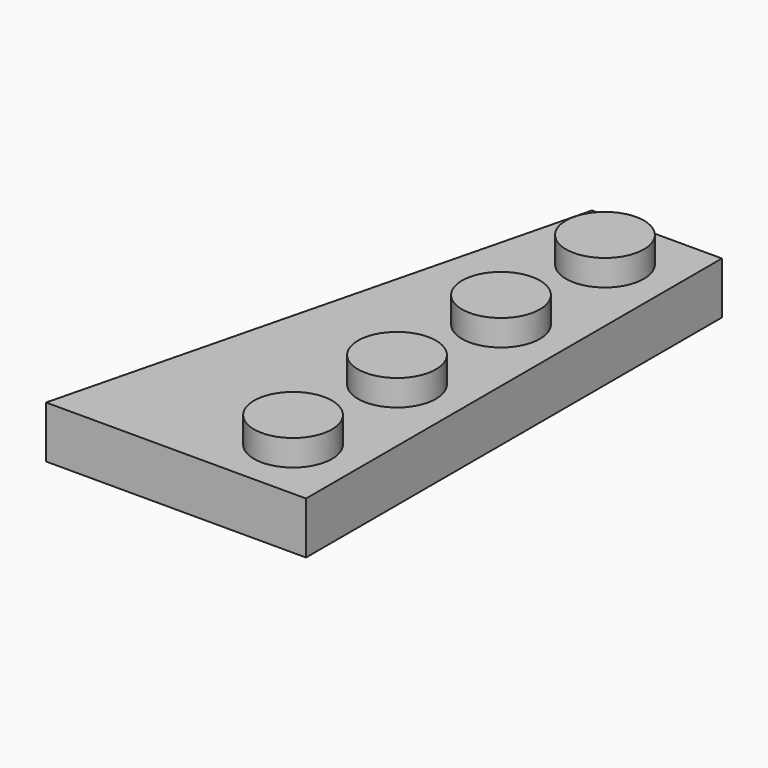
from build123d import *

# Parameters (mm, degrees)
F0_R     = 2.38125
F1_DEPTH = 3.175
F2_DEPTH = 4.7625
F3_T     = -1.5875
F4_R     = 3.175
F4_R_2   = 2.38125
F5_DEPTH = 1.5875


with BuildPart() as f1:
    # F0 (on Top) → F1 (new body)
    with BuildSketch(Plane.XY):
        Polygon((7.9375, 15.875), (0, 15.875), (-7.9375, -15.875), (7.9375, -15.875), align=None)
        with Locations((3.96875, -11.90625)):
            Circle(F0_R, mode=Mode.SUBTRACT)
        with Locations((3.96875, -3.96875)):
            Circle(F0_R, mode=Mode.SUBTRACT)
        with Locations((3.96875, 3.96875)):
            Circle(F0_R, mode=Mode.SUBTRACT)
        with Locations((3.96875, 11.90625)):
            Circle(F0_R, mode=Mode.SUBTRACT)
    extrude(amount=F1_DEPTH)

    # F0 (on Top) → F2 (join)
    with BuildSketch(Plane.XY):
        with Locations((3.96875, 11.90625)):
            Circle(F0_R)
        with Locations((3.96875, 3.96875)):
            Circle(F0_R)
        with Locations((3.96875, -3.96875)):
            Circle(F0_R)
        with Locations((3.96875, -11.90625)):
            Circle(F0_R)
    extrude(amount=F2_DEPTH)

    # F3
    f3_openings = [f1.faces().sort_by_distance(p)[0] for p in [
        (1.763889, -1.763889, 0),
    ]]
    offset(amount=F3_T, openings=f3_openings, kind=Kind.INTERSECTION)

    # F4 (on face) → F5 (join)
    with BuildSketch(Plane(origin=(0, 0, 1.5875), x_dir=(1, 0, 0), z_dir=(0, 0, -1))):
        with BuildLine():
            ThreePointArc((0.4381385265, -11.0821239253), (2.3949650124, -10.0219106095), (3.175, -7.9375))
            ThreePointArc((3.175, -7.9375), (1.8179135149, -5.3344603437), (-1.0932302062, -4.9566489946))
            Line((-1.0932302062, -4.9566489946), (-0.8992491716, -5.7325731328))
            ThreePointArc((-0.8992491716, -5.7325731328), (1.3283475585, -5.9611790933), (2.38125, -7.9375))
            ThreePointArc((2.38125, -7.9375), (1.7680146479, -9.5326413001), (0.244157492, -10.3061997871))
            Line((0.244157492, -10.3061997871), (0.4381385265, -11.0821239253))
        make_face()
        with BuildLine():
            Line((-2.0152745824, -1.2684714896), (-1.6550091801, -2.7095330988))
            ThreePointArc((-1.6550091801, -2.7095330988), (1.5533787132, -2.7690503017), (3.175, 0))
            ThreePointArc((3.175, 0), (0.8354053628, 3.0631230599), (-2.7353766172, 1.6119366495))
            Line((-2.7353766172, 1.6119366495), (-2.3751112149, 0.1708750402))
            ThreePointArc((-2.3751112149, 0.1708750402), (0.0854926372, 2.3797148089), (2.38125, 0))
            ThreePointArc((2.38125, 0), (0.6601056594, -2.2879274641), (-2.0152745824, -1.2684714896))
        make_face()
        with Locations((0, 7.9375)):
            Circle(F4_R)
        with Locations((0, 7.9375)):
            Circle(F4_R_2, mode=Mode.SUBTRACT)
    extrude(amount=F5_DEPTH)


solid = f1.part
